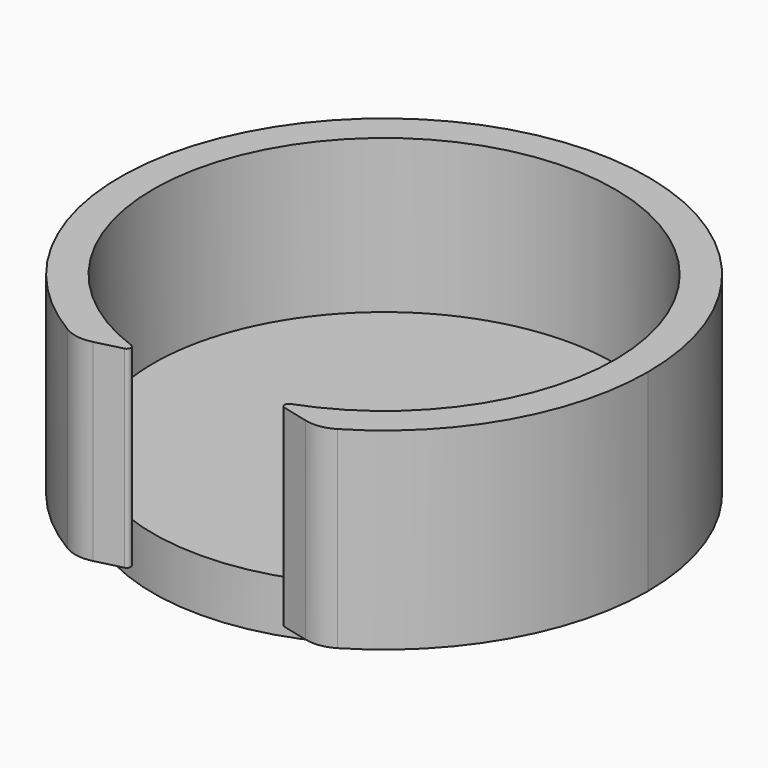
from build123d import *

# Parameters (mm, degrees)
F1_DEPTH = 30.5
F2_F1_R  = 0.65
F2_F2_R  = 0.65
F3_R     = 6
F4_DEPTH = 6.28
F5_DEPTH = 2


with BuildPart() as f1:
    # F0 (on Top) → F1 (new body)
    with BuildSketch(Plane.XY):
        with BuildLine():
            ThreePointArc((19.1, -37.1079536623), (35.6296837272, -21.7332892701), (41.735, 0))
            ThreePointArc((41.735, 0), (-21.7332892701, 35.6296837272), (-19.1, -37.1079536623))
            Line((-19.1, -37.1079536623), (-10.5, -34.9571165859))
            ThreePointArc((-10.5, -34.9571165859), (-21.7830209108, 29.2873692912), (36.5, 0))
            ThreePointArc((36.5, 0), (29.2873692912, -21.7830209108), (10.5, -34.9571165859))
            Line((10.5, -34.9571165859), (19.1, -37.1079536623))
        make_face()
    extrude(amount=F1_DEPTH)

    # F2: fillet of radius 0.65 on 2 edges, made by hand

    # F2_f1
    f2_f1_edges = [f1.edges().sort_by_distance(p)[0] for p in [
        (10.5, -34.9571165859, 15.25),
    ]]
    fillet(f2_f1_edges, radius=F2_F1_R)

    # F2_f2
    f2_f2_edges = [f1.edges().sort_by_distance(p)[0] for p in [
        (-10.5, -34.9571165859, 15.25),
    ]]
    fillet(f2_f2_edges, radius=F2_F2_R)

    # F3
    f3_edges = [f1.edges().sort_by_distance(p)[0] for p in [
        (-19.1, -37.107954, 15.25),
        (19.1, -37.107954, 15.25),
    ]]
    fillet(f3_edges, radius=F3_R)


with BuildPart() as f4:
    # F0 (on Top) → F4 (new body)
    with BuildSketch(Plane.XY):
        with BuildLine():
            ThreePointArc((36.5, 0), (-21.7830209108, 29.2873692912), (-10.5, -34.9571165859))
            Line((-10.5, -34.9571165859), (0, 0))
            Line((0, 0), (10.5, -34.9571165859))
            ThreePointArc((10.5, -34.9571165859), (29.2873692912, -21.7830209108), (36.5, 0))
        make_face()
        with BuildLine():
            Line((0, 0), (-10.5, -34.9571165859))
            ThreePointArc((-10.5, -34.9571165859), (0, -36.5), (10.5, -34.9571165859))
            Line((10.5, -34.9571165859), (0, 0))
        make_face()
    extrude(amount=F4_DEPTH)

    # F5 (add): a face of the model
    f5_faces = [f4.faces().sort_by_distance(p)[0] for p in [
        (0, 0, 0),
    ]]
    extrude(f5_faces, amount=F5_DEPTH)


solid = Compound([f1.part, f4.part])
